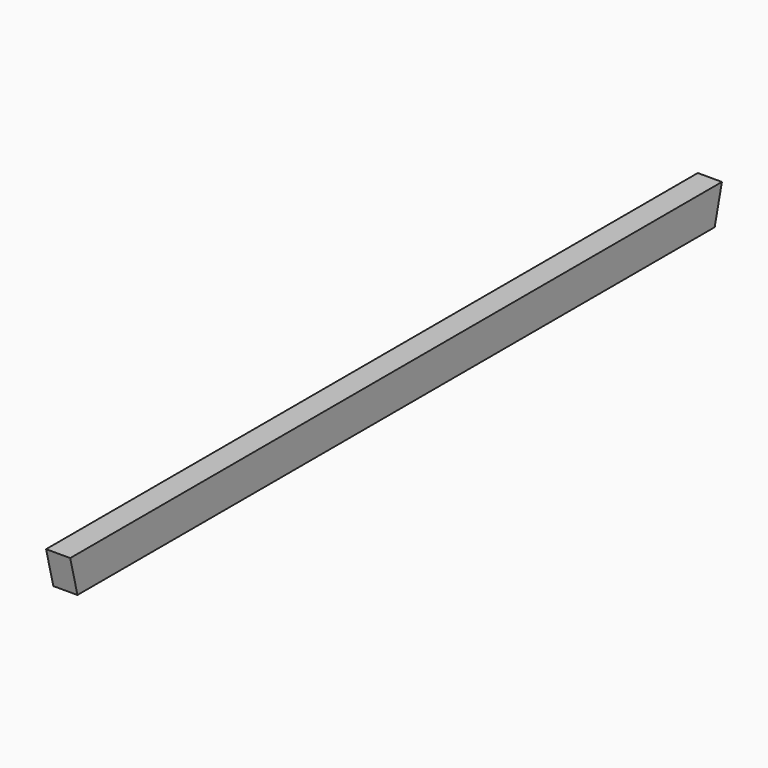
from build123d import *

# Parameters (mm, degrees)
F0_W     = 80
F0_H     = 120
F1_DEPTH = 2700
F2_SIZE2 = 29.99999
F2_SIZE  = 119.99999
F3_SIZE2 = 119.99999
F3_SIZE  = 29.99999


# Not quite as in the source:
# - a fillet or chamfer is up to 0.001 mm smaller than in the source, because OpenCascade refuses the exact size


with BuildPart() as f1:
    # F0 (on Front) → F1 (new body)
    with BuildSketch(Plane.XZ):
        with Locations((40, 60)):
            Rectangle(F0_W, F0_H)
    extrude(amount=-F1_DEPTH)

    # F2 (size 120 and 30 in the source; OpenCascade refuses exactly that, so slightly less here)
    f2_edges = [f1.edges().sort_by_distance(p)[0] for p in [
        (40, 0, 0),
    ]]
    f2_side = f1.faces().sort_by_distance((40, 0, 60))[0]
    chamfer(f2_edges, length=F2_SIZE, length2=F2_SIZE2, reference=f2_side)

    # F3 (size 30 and 120 in the source; OpenCascade refuses exactly that, so slightly less here)
    f3_edges = [f1.edges().sort_by_distance(p)[0] for p in [
        (40, 2700, 0),
    ]]
    f3_side = f1.faces().sort_by_distance((40, 1364.999995, 0))[0]
    chamfer(f3_edges, length=F3_SIZE, length2=F3_SIZE2, reference=f3_side)


solid = f1.part
